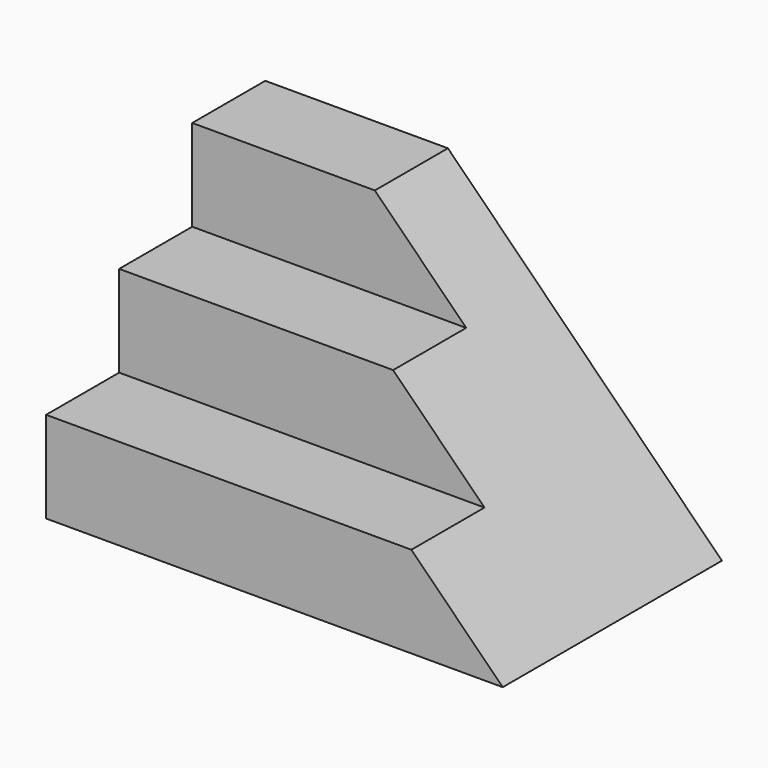
from build123d import *

# Parameters (mm, degrees)
F1_DEPTH = 100
F2_SIZE  = 59.99999


# Not quite as in the source:
# - a fillet or chamfer is up to 0.001 mm smaller than in the source, because OpenCascade refuses the exact size


with BuildPart() as f1:
    # F0 (on Right) → F1 (new body)
    with BuildSketch(Plane.YZ):
        Polygon((-60, 0), (0, 0), (0, 60), (-20, 60), (-20, 40), (-40, 40), (-40, 20), (-60, 20), align=None)
    extrude(amount=F1_DEPTH)

    # F2 (size 60 in the source; OpenCascade refuses exactly that, so slightly less here)
    f2_edges = [f1.edges().sort_by_distance(p)[0] for p in [
        (100, -10, 60),
    ]]
    chamfer(f2_edges, length=F2_SIZE)


solid = f1.part
